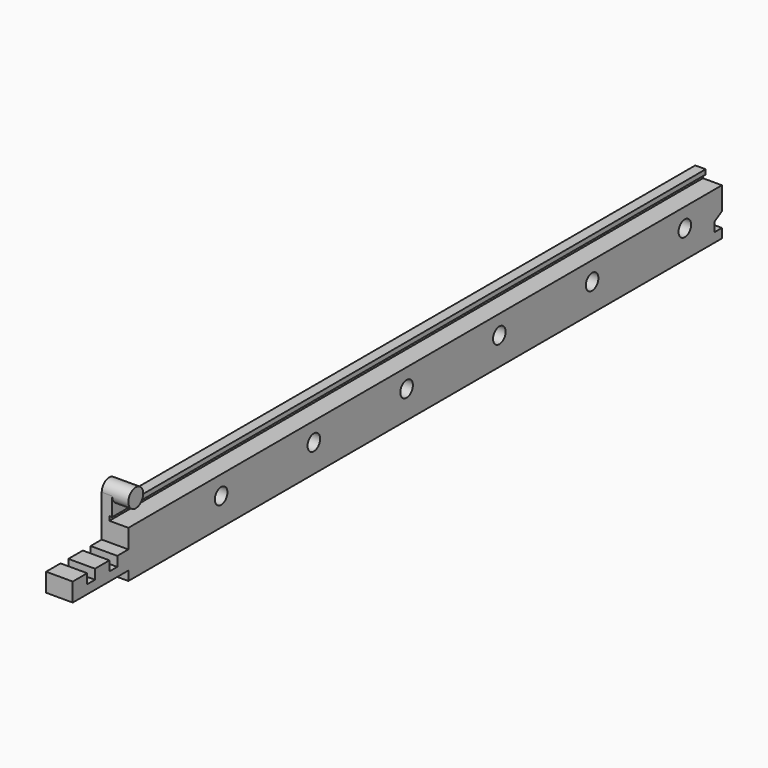
from build123d import *

# Parameters (mm, degrees)
F1_DEPTH  = 5.75
F2_W      = 160
F2_H      = 0.9
F3_DEPTH  = 4.1
F5_DEPTH  = 3.5
F6_R      = 1.7
F7_DEPTH  = 25
F8_R      = 2.85
F8_R_2    = 1.7
F9_DEPTH  = 3
F11_DEPTH = 3.5
F12_W     = 2
F12_H     = 160
F12_W_2   = 3.75
F13_DEPTH = 2
F15_DEPTH = 5.75
F17_DEPTH = 25


# Not quite as in the source:
# - a feature names something its author has since deleted; it is built from what else it names


with BuildPart() as f1:
    # F0 (on Right) → F1 (new body)
    with BuildSketch(Plane.YZ):
        Polygon((-156, 10), (-160, 10), (-160, 0), (0, 0), (0, 10), align=None)
        with BuildLine():
            Line((-160, 13), (-160, 10))
            Line((-160, 10), (-156, 10))
            Line((-156, 10), (-156, 13))
            ThreePointArc((-156, 13), (-156.5857864376, 14.4142135624), (-158, 15))
            ThreePointArc((-158, 15), (-159.4142135624, 14.4142135624), (-160, 13))
        make_face()
    extrude(amount=F1_DEPTH)

    # F2 (on face) → F3 (cut)
    with BuildSketch(Plane.YZ.offset(5.75)):
        with Locations((-80, 8.55)):
            Rectangle(F2_W, F2_H)
    extrude(amount=-F3_DEPTH, mode=Mode.SUBTRACT)

    # F4 (on face) → F5 (cut)
    with BuildSketch(Plane.YZ.offset(5.75)):
        with BuildLine():
            ThreePointArc((-156, 13), (-158, 15), (-160, 13))
            Line((-160, 13), (-160, 9))
            Line((-160, 9), (0, 9))
            Line((0, 9), (0, 10))
            Line((0, 10), (-156, 10))
            Line((-156, 10), (-156, 13))
        make_face()
    extrude(amount=-F5_DEPTH, mode=Mode.SUBTRACT)

    # F6 (on face) → F7 (cut)
    with BuildSketch(Plane(origin=(0, 0, 0), x_dir=(0, -1, 0), z_dir=(-1, 0, 0))):
        with Locations((135, 4)):
            Circle(F6_R)
        with Locations((110, 4)):
            Circle(F6_R)
        with Locations((85, 4)):
            Circle(F6_R)
        with Locations((60, 4)):
            Circle(F6_R)
        with Locations((35, 4)):
            Circle(F6_R)
        with Locations((10, 4)):
            Circle(F6_R)
    extrude(amount=-F7_DEPTH, mode=Mode.SUBTRACT)

    # F8 (on face) → F9 (cut)
    with BuildSketch(Plane(origin=(0, 0, 0), x_dir=(0, -1, 0), z_dir=(-1, 0, 0))):
        with Locations((135, 4)):
            Circle(F8_R)
        with Locations((135, 4)):
            Circle(F8_R_2, mode=Mode.SUBTRACT)
        with Locations((110, 4)):
            Circle(F8_R)
        with Locations((110, 4)):
            Circle(F8_R_2, mode=Mode.SUBTRACT)
        with Locations((85, 4)):
            Circle(F8_R)
        with Locations((85, 4)):
            Circle(F8_R_2, mode=Mode.SUBTRACT)
        with Locations((60, 4)):
            Circle(F8_R)
        with Locations((60, 4)):
            Circle(F8_R_2, mode=Mode.SUBTRACT)
        with Locations((35, 4)):
            Circle(F8_R)
        with Locations((35, 4)):
            Circle(F8_R_2, mode=Mode.SUBTRACT)
        with Locations((10, 4)):
            Circle(F8_R)
        with Locations((10, 4)):
            Circle(F8_R_2, mode=Mode.SUBTRACT)
    extrude(amount=-F9_DEPTH, mode=Mode.SUBTRACT)

    # F10 (on face) → F11 (join, through all)
    with BuildSketch(Plane.YZ.offset(2.25)):
        with BuildLine():
            ThreePointArc((-160, 13), (-158, 11), (-156, 13))
            ThreePointArc((-156, 13), (-158, 15), (-160, 13))
        make_face()
    extrude(amount=F11_DEPTH)

    # F12 (on face) → F13 (join)
    with BuildSketch(Plane(origin=(0, 0, 0), x_dir=(1, 0, 0), z_dir=(0, 0, -1))):
        with Locations((1, 80)):
            Rectangle(F12_W, F12_H)
        with Locations((3.875, 80)):
            Rectangle(F12_W_2, F12_H)
    extrude(amount=F13_DEPTH)

    # F14 (on face) → F15 (join, through all)
    with BuildSketch(Plane.YZ.offset(5.75)):
        Polygon((-175, 0), (-160, 0), (-160, 4), (-163, 4), (-163, 1.9), (-165.1, 1.9), (-165.1, 4), (-169, 4), (-169, 1.9), (-171.1, 1.9), (-171.1, 4), (-175, 4), align=None)
    extrude(amount=-F15_DEPTH)

    # F16 (on face) → F17 (cut)
    with BuildSketch(Plane.YZ.offset(5.75)):
        Polygon((-2, 0), (0, 0), (0, 3.1547005384), (-2, 2), align=None)
    extrude(amount=-F17_DEPTH, mode=Mode.SUBTRACT)


solid = f1.part
